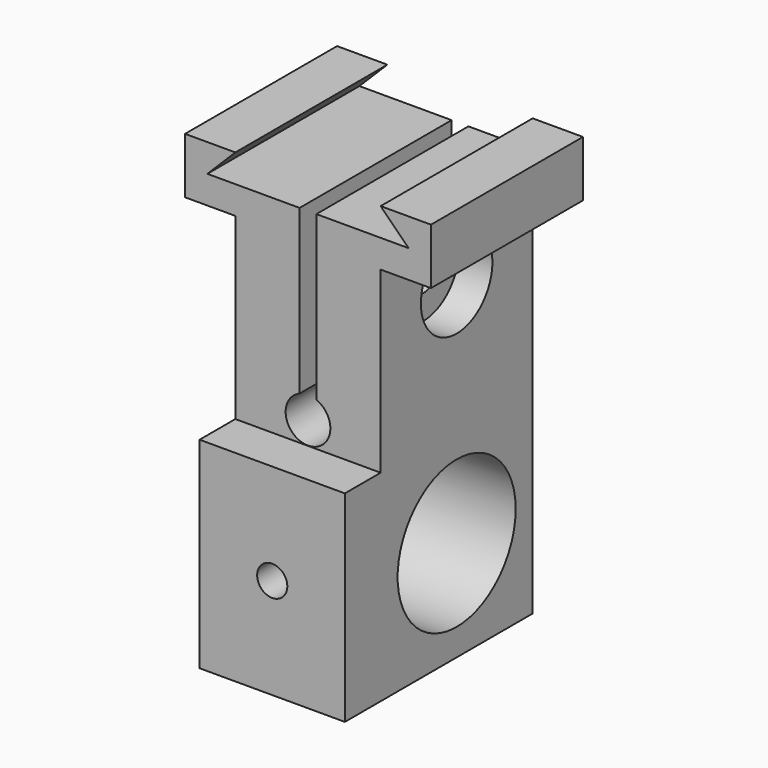
from build123d import *

# Parameters (mm, degrees)
F1_DEPTH  = 21
F2_W      = 22
F2_H      = 21
F3_DEPTH  = 4
F4_R      = 6.6
F4_R_2    = 1.35
F5_DEPTH  = 17.501
F6_R      = 1.8
F7_DEPTH  = 7
F8_R      = 4
F9_DEPTH  = 3
F10_R     = 1.35
F11_DEPTH = 12


# Not quite as in the source:
# - a feature names something its author has since deleted; it is built from what else it names


with BuildPart() as f1:
    # F0 (on Front) → F1 (new body)
    with BuildSketch(Plane.XZ):
        with BuildLine():
            Line((-9, -2.5), (-6.5, 0))
            Line((-6.5, 0), (-11, 0))
            Line((-11, 0), (-11, -5))
            Line((-11, -5), (-6.5, -5))
            Line((-6.5, -5), (-6.5, -39))
            Line((-6.5, -39), (6.5, -39))
            Line((6.5, -39), (6.5, -5))
            Line((6.5, -5), (11, -5))
            Line((11, -5), (11, 0))
            Line((11, 0), (6.5, 0))
            Line((6.5, 0), (9, -2.5))
            Line((9, -2.5), (0.75, -2.5))
            Line((0.75, -2.5), (0.75, -17.11916493))
            ThreePointArc((0.75, -17.11916493), (0, -20.9732145518), (-0.75, -17.11916493))
            Line((-0.75, -17.11916493), (-0.75, -2.5))
            Line((-0.75, -2.5), (-9, -2.5))
        make_face()
    extrude(amount=F1_DEPTH)

    # F2 (on face) → F3 (cut)
    with BuildSketch(Plane.XZ.offset(21)):
        with Locations((0, -10.5)):
            Rectangle(F2_W, F2_H)
    extrude(amount=-F3_DEPTH, mode=Mode.SUBTRACT)

    # F4 (on face) → F5 (cut, through all)
    with BuildSketch(Plane.YZ.offset(6.5)):
        with Locations((-8.5, -30)):
            Circle(F4_R)
        with Locations((-8.5, -9.5)):
            Circle(F4_R_2)
    extrude(amount=-F5_DEPTH, mode=Mode.SUBTRACT)

    # F6 (on face) → F7 (cut)
    with BuildSketch(Plane.YZ.offset(6.5)):
        with Locations((-8.5, -9.5)):
            Circle(F6_R)
    extrude(amount=-F7_DEPTH, mode=Mode.SUBTRACT)

    # F8 (on face) → F9 (cut)
    with BuildSketch(Plane.YZ.offset(6.5)):
        with Locations((-8.5, -9.5)):
            Circle(F8_R)
    extrude(amount=-F9_DEPTH, mode=Mode.SUBTRACT)

    # F10 (on face) → F11 (cut)
    with BuildSketch(Plane.XZ.offset(21)):
        with Locations((0, -30)):
            Circle(F10_R)
    extrude(amount=-F11_DEPTH, mode=Mode.SUBTRACT)


solid = f1.part
